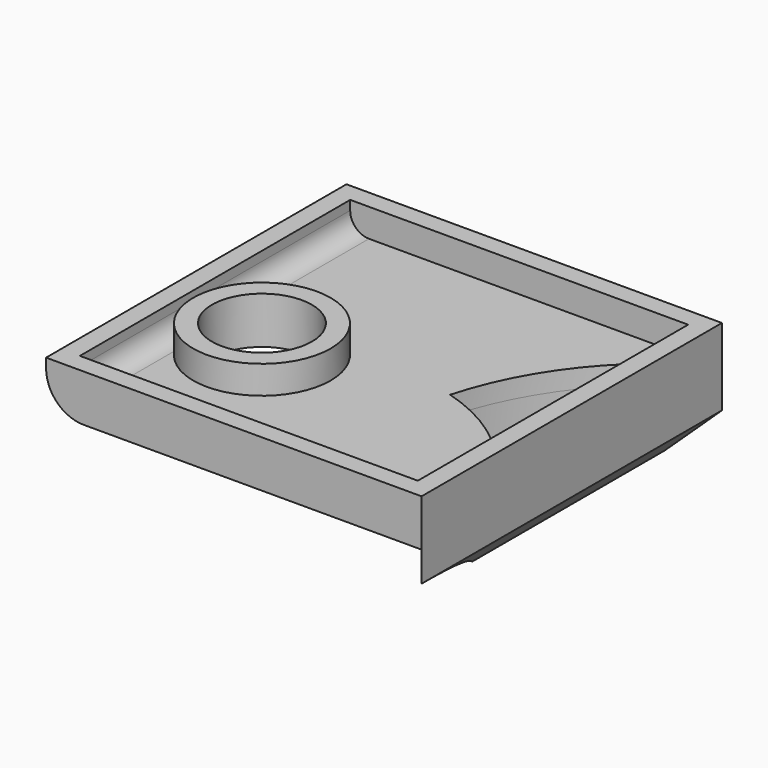
from build123d import *

# Parameters (mm, degrees)
F0_W        = 50.8
F0_H        = 50.8
F1_DEPTH    = 6.35
F3_DEPTH    = 9.144
F2_R        = 6.7603485979
F4_DEPTH    = 25.4
F5_R        = 5.08
F6_T1_DEPTH = 86.0732038629
F7_T        = 2.54
F7_T4_ANGLE = 49.6458001059
F7_T6_ANGLE = 79.2883730852


# Not quite as in the source:
# - a fillet or chamfer that OpenCascade refuses, or shapes differently, is made with other operations: its cross-section is extruded or revolved along the edge and cut away or added
# - a shell that OpenCascade refuses in one call is made with other operations: the cavity is built on its own and cut out


with BuildPart() as f1:
    # F0 (on Top) → F1 (new body)
    with BuildSketch(Plane.XY):
        with Locations((-25.4, 25.4)):
            Rectangle(F0_W, F0_H)
    extrude(amount=-F1_DEPTH)

    # F2 (on face) → F3 (join)
    with BuildSketch(Plane(origin=(0, 0, -6.35), x_dir=(1, 0, 0), z_dir=(0, 0, -1))):
        with BuildLine():
            ThreePointArc((0, 0), (-5.5886686099, -15.504363354), (-19.7841264307, -23.8773841411))
            ThreePointArc((-19.7841264307, -23.8773841411), (-12.8545439956, -39.5156757118), (0, -50.8))
            Line((0, -50.8), (0, 0))
        make_face()
    extrude(amount=F3_DEPTH)

    # F2 (on face) → F4 (cut)
    with BuildSketch(Plane(origin=(0, 0, -6.35), x_dir=(1, 0, 0), z_dir=(0, 0, -1))):
        with Locations((-37.9167422652, -20.3997846693)):
            Circle(F2_R)
    extrude(amount=-F4_DEPTH, mode=Mode.SUBTRACT)

    # F5
    f5_edges = [f1.edges().sort_by_distance(p)[0] for p in [
        (-50.8, 25.4, -6.35),
    ]]
    fillet(f5_edges, radius=F5_R)

    # F6: chamfer of 5.08 on 1 edges, made by hand

    # F6_s2 → F6_t1 (cut)
    with BuildSketch(Plane.XZ.offset(-63.8641495789)):
        Polygon((0, -10.414), (-5.08, -15.494), (0, -15.494), align=None)
    extrude(amount=F6_T1_DEPTH, mode=Mode.SUBTRACT)

    # F7: shell of thickness 2.54, made by hand


with BuildPart() as f7_core1:
    # F7_t2: copy of F1
    add(f1.part)

    # the walls: a layer under each face that stays
    f7_faces = [f7_core1.faces().sort_by_distance(p)[0] for p in [
        (-25.4, 0, -3.175),
        (-50.8, 25.4, -0.635),
        (-49.3121024484, 25.4, -4.8621024484),
        (-22.86, 25.4, -6.35),
        (0, 25.4, -5.207),
        (-25.4, 50.8, -3.175),
        (-44.6770908632, 20.3997846693, -3.175),
        (-12.8545439956, 39.5156757118, -10.922),
        (-5.5886686099, 15.504363354, -10.922),
        (-2.54, 25.4, -12.954),
        (-12.4320632154, 31.169630086, -15.494),
    ]]
    thicken(f7_faces, amount=-F7_T, mode=Mode.SUBTRACT)

    # F7_s3 → F7_t4 (revolve, cut)
    with BuildSketch(Plane(origin=(3.8753287702, 19.0692040386, 0), x_dir=(0, 0, 1), z_dir=(-0.1991535327, -0.9799683007, 0))):
        Polygon((-6.3754, 24.1684821625), (-3.81, 24.1430821625), (-3.81, 21.6030821625), (-6.35, 21.6030821625), align=None)
    revolve(axis=Axis((19.2103228569, 15.9527580845, -6.35), (0, 0, -1)), revolution_arc=F7_T4_ANGLE, mode=Mode.SUBTRACT)

    # F7_s5 → F7_t6 (revolve, cut)
    with BuildSketch(Plane.XZ):
        Polygon((-0.0254, -6.3754), (0, -3.81), (2.54, -3.81), (2.54, -6.35), align=None)
    revolve(axis=Axis((-24.3008235773, 0, -6.35), (0, 0, 1)), revolution_arc=F7_T6_ANGLE, mode=Mode.SUBTRACT)


with BuildPart() as f1_1:
    add(f1.part)

    # what is left inside the walls is the cavity
    f7_cavity = [f7_core1.part.solids().sort_by_distance(p)[0] for p in [
        (-25.4, 17.78, -0.0254),
    ]]
    add(f7_cavity, mode=Mode.SUBTRACT)


solid = f1_1.part
